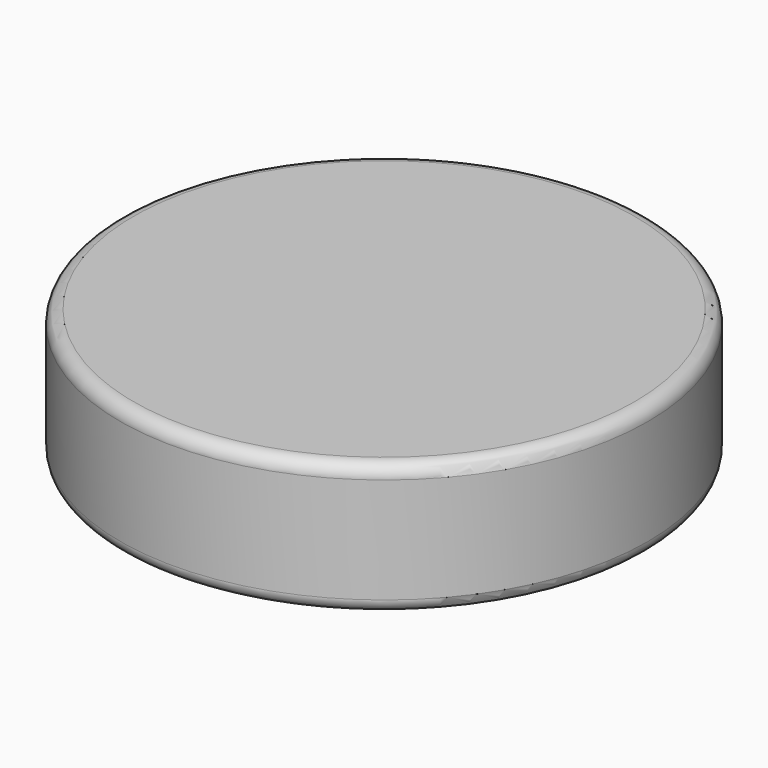
from build123d import *

# Parameters (mm, degrees)
F0_R     = 20
F1_DEPTH = 10
F3_R     = 1
F4_R     = 1


# Not quite as in the source:
# - the program builds the solid bodies; features that only make, move or delete a surface that nothing else refers to are left out


with BuildPart() as f1:
    # F0 (on Top) → F1 (new body)
    with BuildSketch(Plane.XY):
        Circle(F0_R)
    extrude(amount=F1_DEPTH)

    # F3
    f3_edges = [f1.edges().sort_by_distance(p)[0] for p in [
        (-20, 0, 0),
    ]]
    fillet(f3_edges, radius=F3_R)

    # F4
    f4_edges = [f1.edges().sort_by_distance(p)[0] for p in [
        (-20, 0, 10),
    ]]
    fillet(f4_edges, radius=F4_R)


solid = f1.part
